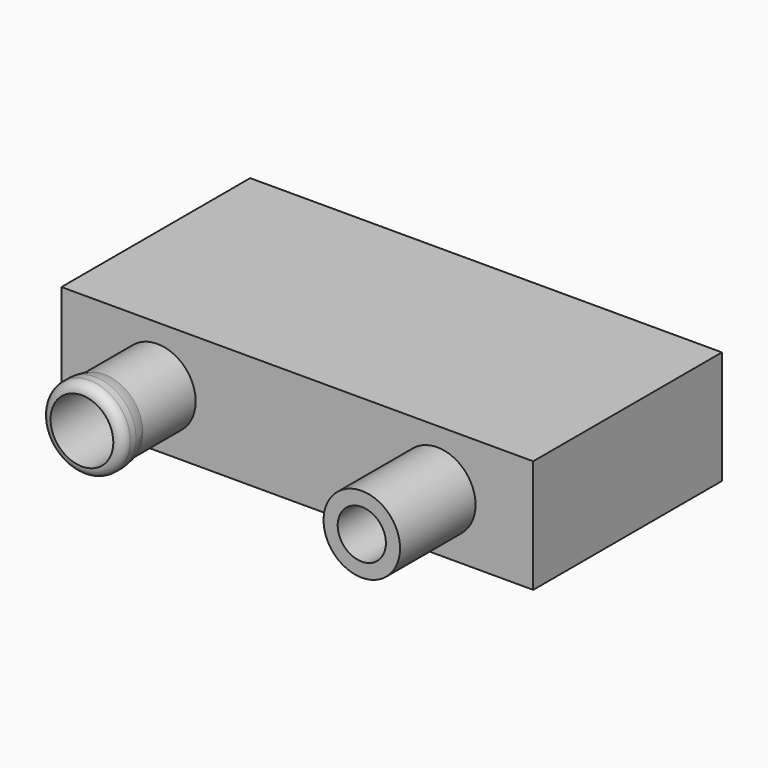
from build123d import *

# Parameters (mm, degrees)
F0_W     = 50
F0_H     = 25
F1_DEPTH = 12
F2_R     = 4.0545181675
F3_DEPTH = 10
F4_T     = -1.5
F5_R     = 4.327746069
F6_DEPTH = 3
F8_R     = 1
F9_DEPTH = 20


# Not quite as in the source:
# - a fillet or chamfer that OpenCascade refuses, or shapes differently, is made with other operations: its cross-section is extruded or revolved along the edge and cut away or added


with BuildPart() as f1:
    # F0 (on Top) → F1 (new body)
    with BuildSketch(Plane.XY):
        Rectangle(F0_W, F0_H)
    extrude(amount=F1_DEPTH)

    # F2 (on face) → F3 (join)
    with BuildSketch(Plane.XZ.offset(12.5)):
        with Locations((-14.8313278332, 5.9491097927)):
            Circle(F2_R)
        with Locations((14.8313278332, 5.9491097927)):
            Circle(F2_R)
    extrude(amount=F3_DEPTH)

    # F4
    f4_openings = [f1.faces().sort_by_distance(p)[0] for p in [
        (14.831328, -22.5, 5.94911),
        (-14.831328, -22.5, 5.94911),
    ]]
    offset(amount=F4_T, openings=f4_openings, kind=Kind.INTERSECTION)

    # F5 (on face) → F6 (join)
    with BuildSketch(Plane.XZ.offset(22.5)):
        with Locations((-14.8313278332, 5.9491097927)):
            Circle(F5_R)
    extrude(amount=-F6_DEPTH)

    # F7: fillet of radius 3 on 1 edges, made by hand

    # F7_s1 → F7_t2 (revolve, cut)
    with BuildSketch(Plane.XY.offset(5.9491097927)):
        with BuildLine():
            ThreePointArc((-10.7768096658, -19.5), (-10.5726846068, -20.1106963365), (-10.5035817643, -20.7508852557))
            Line((-10.5035817643, -20.7508852557), (-10.5035817643, -19.5))
            Line((-10.5035817643, -19.5), (-10.7768096658, -19.5))
        make_face()
    revolve(axis=Axis((-14.8313278332, -19.5, 5.9491097927), (0, -1, 0)), mode=Mode.SUBTRACT)

    # F8
    f8_edges = [f1.edges().sort_by_distance(p)[0] for p in [
        (-19.159074, -22.5, 5.94911),
    ]]
    fillet(f8_edges, radius=F8_R)

    # F9 (cut): a face of the model
    f9_faces = [f1.faces().sort_by_distance(p)[0] for p in [
        (-14.8313278332, -22.5, 5.9491097927),
    ]]
    extrude(f9_faces, amount=-F9_DEPTH, mode=Mode.SUBTRACT)


solid = f1.part
